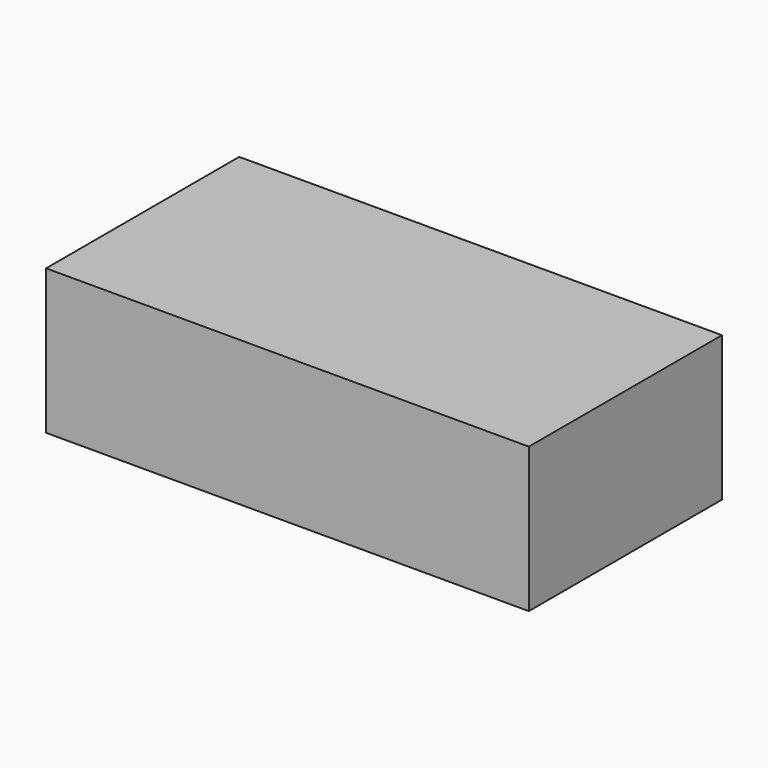
from build123d import *

# Parameters (mm, degrees)
F0_W     = 50
F0_H     = 15
F1_DEPTH = 25


# Not quite as in the source:
# - the program builds the solid bodies; features that only make, move or delete a surface that nothing else refers to are left out


with BuildPart() as f1:
    # F0 (on Front) → F1 (new body)
    with BuildSketch(Plane.XZ):
        with Locations((25, 7.5)):
            Rectangle(F0_W, F0_H)
    extrude(amount=F1_DEPTH)


solid = f1.part
